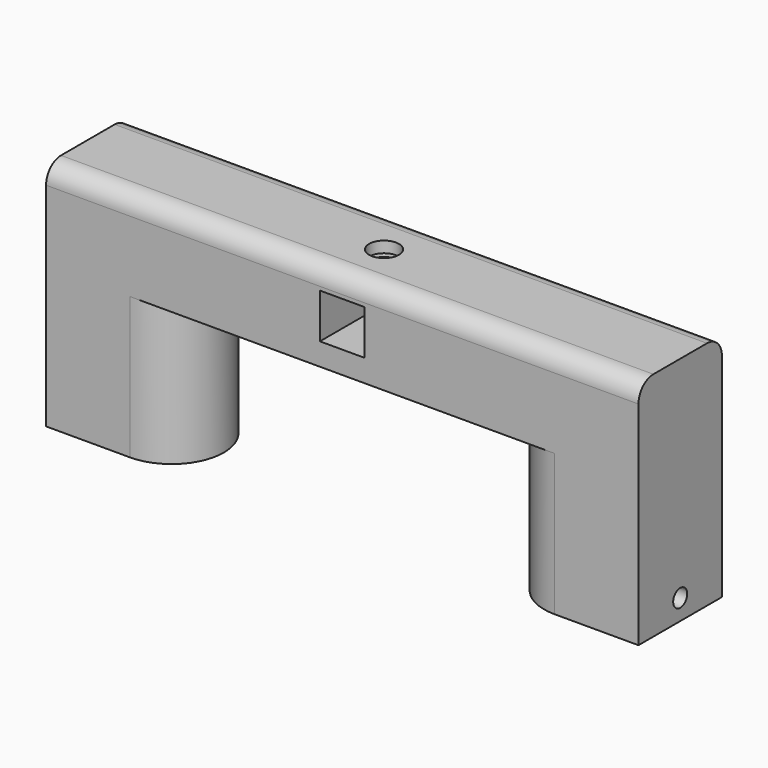
from build123d import *

# Parameters (mm, degrees)
F0_W            = 12
F0_H            = 12
F1_DEPTH        = 28
F2_DEPTH        = 4
F3_W            = 2.4
F3_H            = 13
F4_DEPTH        = 13
F5_R            = 2.35
F6_DEPTH        = 14.5
F9_DEPTH        = 38
F11_D           = 4.8
F11_CBORE_D     = 8
F11_CBORE_DEPTH = 3
F12_DEPTH       = 4
F13_R           = 5


# Not quite as in the source:
# - a pattern or mirror of a feature is missing from the dataset's text; its kind, count and spacing are read off the source's solid


with BuildPart() as f1:
    # F0 (on Front) → F1 (new body)
    with BuildSketch(Plane.XZ):
        Polygon((0, 62), (0, 0), (14.5, 0), (14.5, 38), (144.5, 38), (144.5, 0), (159, 0), (159, 62), align=None)
        with Locations((79.5, 50)):
            Rectangle(F0_W, F0_H, mode=Mode.SUBTRACT)
    extrude(amount=F1_DEPTH)

    # F0 (on Front) → F2 (join)
    with BuildSketch(Plane.XZ):
        with Locations((79.5, 50)):
            Rectangle(F0_W, F0_H)
    extrude(amount=F2_DEPTH)

    # F3 (on face) → F4 (cut)
    with BuildSketch(Plane(origin=(0, 0, 0), x_dir=(1, 0, 0), z_dir=(0, 0, -1))):
        with Locations((7, 14)):
            Rectangle(F3_W, F3_H)
        with Locations((152, 14)):
            Rectangle(F3_W, F3_H)
    extrude(amount=-F4_DEPTH, mode=Mode.SUBTRACT)

    # F5 (on face) → F6 (cut)
    with BuildSketch(Plane(origin=(0, 0, 0), x_dir=(0, -1, 0), z_dir=(-1, 0, 0))):
        with Locations((14, 5.5)):
            Circle(F5_R)
    f6 = extrude(amount=-F6_DEPTH, mode=Mode.SUBTRACT)

    # F6_copies: F6 across plane
    add(f6.mirror(Plane(origin=(79.5, 0, 0), x_dir=(0, 0, 1), z_dir=(1, 0, 0))), mode=Mode.SUBTRACT)

    # F8 (on face) → F9 (join, through all)
    with BuildSketch(Plane(origin=(0, 0, 38), x_dir=(1, 0, 0), z_dir=(0, 0, -1))):
        with BuildLine():
            ThreePointArc((14.5, 24), (20.5, 14), (14.5, 4))
            Line((14.5, 4), (14.5, 0))
            Line((14.5, 0), (22.5, 0))
            ThreePointArc((22.5, 0), (36.5, 14), (22.5, 28))
            Line((22.5, 28), (14.5, 28))
            Line((14.5, 28), (14.5, 24))
        make_face()
    f9 = extrude(amount=F9_DEPTH)

    # F9_copies: F9 across plane
    add(f9.mirror(Plane(origin=(79.5, 0, 0), x_dir=(0, 0, 1), z_dir=(1, 0, 0))))

    # F11 (through all)
    with Locations(Plane.XY.offset(62)):
        with Locations((79.5, -14)):
            CounterBoreHole(F11_D / 2, F11_CBORE_D / 2, F11_CBORE_DEPTH)

    # F8 (on face) → F12 (cut)
    with BuildSketch(Plane(origin=(0, 0, 38), x_dir=(1, 0, 0), z_dir=(0, 0, -1))):
        Polygon((79.5955098336, 9.4009916426), (83.5306129865, 11.7832097635), (83.4351031529, 16.3822181209), (79.4044901664, 18.5990083574), (75.4693870135, 16.2167902365), (75.5648968471, 11.6177818791), align=None)
    extrude(amount=-F12_DEPTH, mode=Mode.SUBTRACT)

    # F13
    f13_edges = [f1.edges().sort_by_distance(p)[0] for p in [
        (79.5, -28, 62),
        (79.5, 0, 62),
    ]]
    fillet(f13_edges, radius=F13_R)


solid = f1.part
